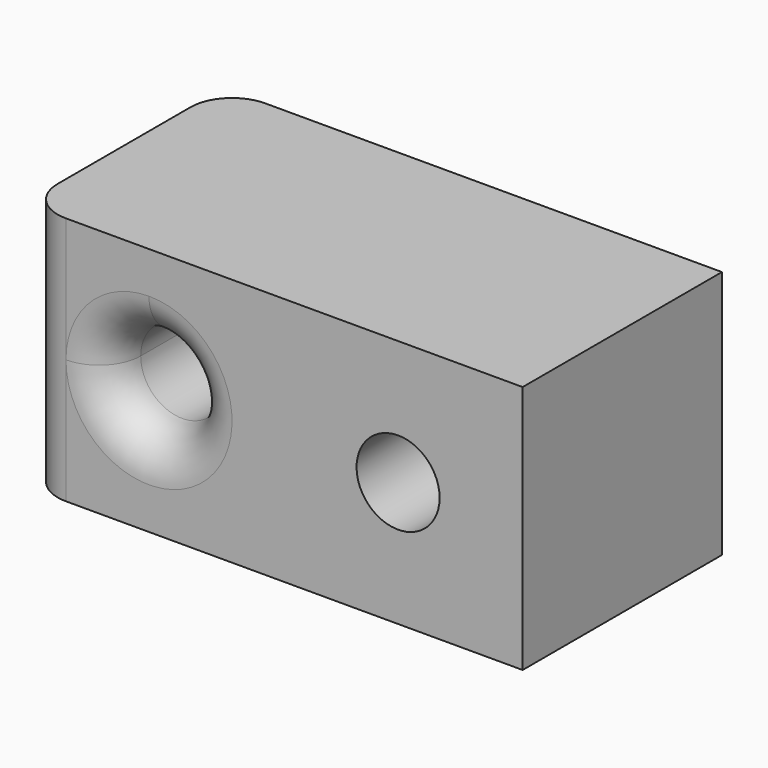
from build123d import *

# Parameters (mm, degrees)
F0_W     = 30
F0_H     = 30
F1_DEPTH = 30
F3_DEPTH = 30.001
F5_R     = 5
F6_R     = 4.99999


# Not quite as in the source:
# - a fillet or chamfer is up to 0.001 mm smaller than in the source, because OpenCascade refuses the exact size


with BuildPart() as f1:
    # F0 (on Top) → F1 (new body)
    with BuildSketch(Plane.XY):
        with Locations((-170.8580559492, -194.9572271109)):
            Rectangle(F0_W, F0_H)
    extrude(amount=F1_DEPTH)

    # F2 (on face) → F3 (cut, through all)
    with BuildSketch(Plane.XZ.offset(209.9572271109)):
        with BuildLine():
            ThreePointArc((-170.8580559492, 20), (-174.3935898551, 11.4644660941), (-165.8580559492, 15))
            ThreePointArc((-165.8580559492, 15), (-167.3225220433, 18.5355339059), (-170.8580559492, 20))
        make_face()
    extrude(amount=-F3_DEPTH, mode=Mode.SUBTRACT)

    # F4: F1 across face


with BuildPart() as f1_1:
    add(f1.part)
    add(f1.part.mirror(Plane(origin=(-185.8580559492, -194.9572271109, 15), x_dir=(0, -1, 0), z_dir=(-1, 0, 0))))

    # F5
    f5_edges = [f1_1.edges().sort_by_distance(p)[0] for p in [
        (-215.858056, -209.957227, 15),
    ]]
    fillet(f5_edges, radius=F5_R)

    # F6 (radius 5 in the source; OpenCascade refuses exactly that, so slightly less here)
    f6_edges = [f1_1.edges().sort_by_distance(p)[0] for p in [
        (-215.858056, -179.957227, 15),
        (-195.858056, -209.957227, 15),
    ]]
    fillet(f6_edges, radius=F6_R)


solid = f1_1.part
